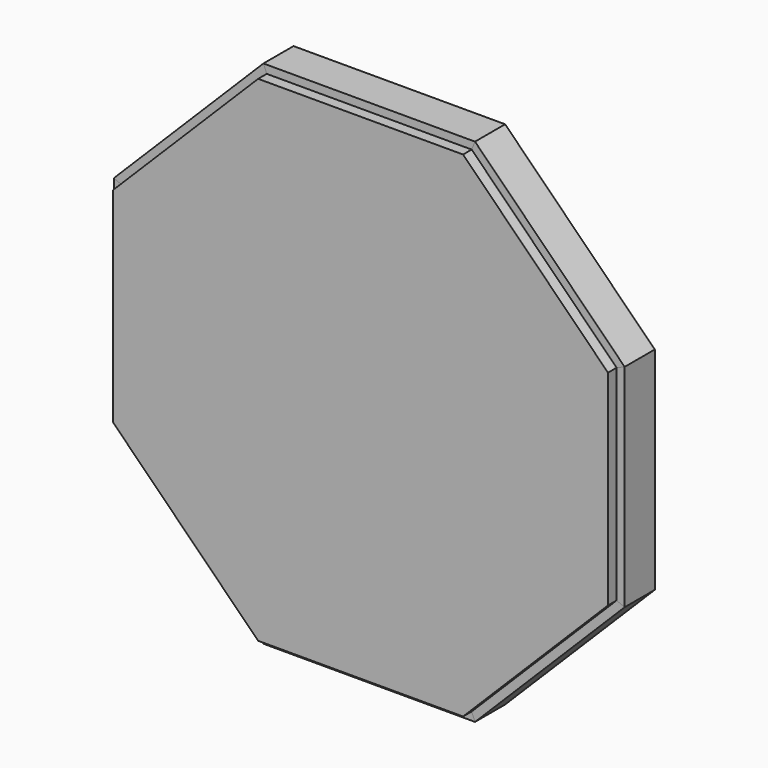
from build123d import *

# Parameters (mm, degrees)
F2_DEPTH      = 50.8
F5_DEPTH      = 38.1
F5_DEPTH_BACK = 6.35
F14_DEPTH     = 6.35


# Not quite as in the source:
# - a variable given as a bare number and used for a length is read in inches; the dataset says mm whatever the document's units were
# - a length typed as a fraction of an inch, garbled in the dataset ("3 / 203.2 mm" for 3/8 in), is restored


with BuildPart() as f2:
    # F1 (on Front) → F2 (new body)
    with BuildSketch(Plane.XZ):
        Polygon((292.0999999997, -120.9917815691), (292.0999999997, 120.9917815691), (120.9917815691, 292.0999999997), (-120.9917815691, 292.0999999997), (-292.0999999997, 120.9917815691), (-292.0999999997, -120.9917815691), (-120.9917815691, -292.0999999997), (120.9917815691, -292.0999999997), align=None)
    extrude(amount=F2_DEPTH)


with BuildPart() as f5:
    # F4 (on Front) → F5 (new body, two sides)
    with BuildSketch(Plane.XZ) as f5_sk:
        Polygon((124.9371657507, 301.6249999997), (-124.9371657507, 301.6249999997), (-120.9917815691, 292.0999999997), (120.9917815691, 292.0999999997), align=None)
    extrude(amount=F5_DEPTH)
    extrude(f5_sk.sketch, amount=-F5_DEPTH_BACK)


with BuildPart() as f6_1:
    # F6: instance of F5
    add(f5.part.mirror(Plane.XY))


with BuildPart() as f7_1:
    # F7: instance of F5
    add(f5.part.mirror(Plane(origin=(122.9644736599, -15.875, 296.8624999997), x_dir=(0, 1, 0), z_dir=(0.9238795325, 0, -0.3826834324))))


with BuildPart() as f8_1:
    # F8: instance of F7_1
    add(f7_1.part.mirror(Plane(origin=(296.8624999997, -15.875, 122.9644736599), x_dir=(1, 0, 0), z_dir=(0.3826834324, 0, -0.9238795325))))


with BuildPart() as f9_1:
    # F9: instance of F8_1
    add(f8_1.part.mirror(Plane(origin=(296.8624999997, -15.875, -122.9644736599), x_dir=(1, 0, 0), z_dir=(-0.3826834324, 0, -0.9238795325))))


with BuildPart() as f10_1:
    # F10: instance of F6_1
    add(f6_1.part.mirror(Plane(origin=(-122.9644736599, -15.875, -296.8624999997), x_dir=(0, -1, 0), z_dir=(-0.9238795325, 0, 0.3826834324))))


with BuildPart() as f11_1:
    # F11: instance of F10_1
    add(f10_1.part.mirror(Plane(origin=(-296.8624999997, -15.875, -122.9644736599), x_dir=(1, 0, 0), z_dir=(-0.3826834324, 0, 0.9238795325))))


with BuildPart() as f12_1:
    # F12: instance of F11_1
    add(f11_1.part.mirror(Plane(origin=(-296.8624999997, -15.875, 122.9644736599), x_dir=(1, 0, 0), z_dir=(0.3826834324, 0, 0.9238795325))))


with BuildPart() as f14:
    # F13 (on face) → F14 (new body)
    with BuildSketch(Plane(origin=(0, 0, 0), x_dir=(-1, 0, 0), z_dir=(0, 1, 0))):
        Polygon((-122.9644736599, -296.8624999997), (122.9644736599, -296.8624999997), (296.8624999997, -122.9644736599), (296.8624999997, 122.9644736599), (122.9644736599, 296.8624999997), (-122.9644736599, 296.8624999997), (-296.8624999997, 122.9644736599), (-296.8624999997, -122.9644736599), align=None)
    extrude(amount=F14_DEPTH)


with BuildPart() as f5_1:
    add(f5.part)

    # F15: cut F14
    add(f14.part, mode=Mode.SUBTRACT)


with BuildPart() as f6_1_1:
    add(f6_1.part)

    # F15: cut F14
    add(f14.part, mode=Mode.SUBTRACT)


with BuildPart() as f7_1_1:
    add(f7_1.part)

    # F15: cut F14
    add(f14.part, mode=Mode.SUBTRACT)


with BuildPart() as f8_1_1:
    add(f8_1.part)

    # F15: cut F14
    add(f14.part, mode=Mode.SUBTRACT)


with BuildPart() as f9_1_1:
    add(f9_1.part)

    # F15: cut F14
    add(f14.part, mode=Mode.SUBTRACT)


with BuildPart() as f10_1_1:
    add(f10_1.part)

    # F15: cut F14
    add(f14.part, mode=Mode.SUBTRACT)


with BuildPart() as f11_1_1:
    add(f11_1.part)

    # F15: cut F14
    add(f14.part, mode=Mode.SUBTRACT)


with BuildPart() as f12_1_1:
    add(f12_1.part)

    # F15: cut F14
    add(f14.part, mode=Mode.SUBTRACT)


solid = Compound([f2.part, f14.part, f5_1.part, f6_1_1.part, f7_1_1.part, f8_1_1.part, f9_1_1.part, f10_1_1.part, f11_1_1.part, f12_1_1.part])
